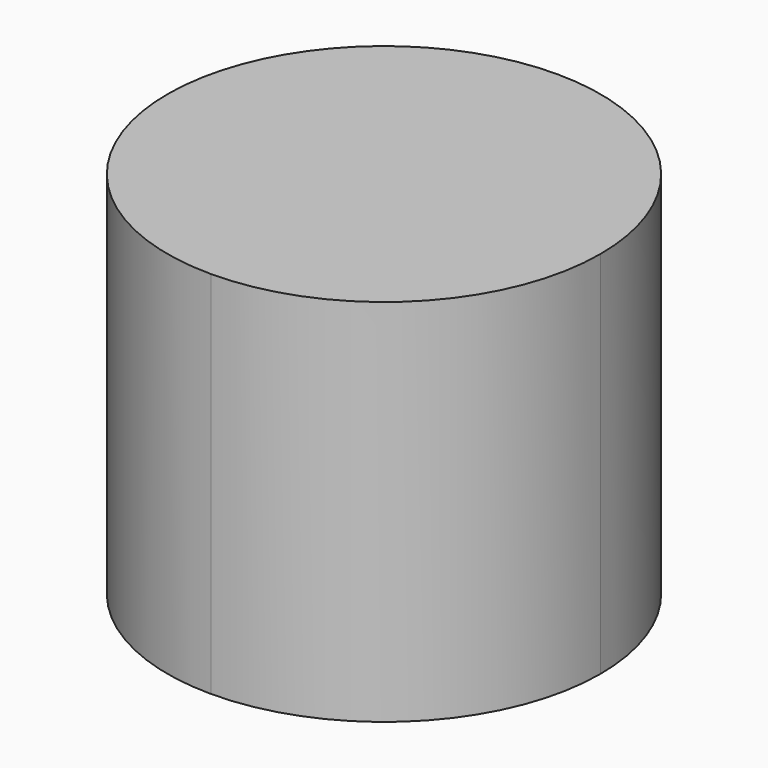
from build123d import *

# Parameters (mm, degrees)
F4_DEPTH = 25.4


# Not quite as in the source:
# - the program builds the solid bodies; features that only make, move or delete a surface that nothing else refers to are left out


with BuildPart() as f4:
    # F2 (on Top) → F4 (new body)
    with BuildSketch(Plane.XY):
        with BuildLine():
            ThreePointArc((0, -14.8716701685), (10.5158588237, -10.5158588237), (14.8716701685, 0))
            ThreePointArc((14.8716701685, 0), (14.0140961938, 4.9771157786), (11.5402781738, 9.3802213871))
            ThreePointArc((11.5402781738, 9.3802213871), (6.390110133, 13.4288147686), (0, 14.8716701685))
            ThreePointArc((0, 14.8716701685), (-6.2616501648, 13.4891923707), (-11.3591281509, 9.598790614))
            ThreePointArc((-11.3591281509, 9.598790614), (-13.9347393829, 5.1951527343), (-14.8705786933, 0.1801747106))
            ThreePointArc((-14.8705786933, 0.1801747106), (-14.0394042685, -4.9052728146), (-11.5226990459, -9.401807289))
            ThreePointArc((-11.5226990459, -9.401807289), (-6.3775385774, -13.4347897377), (0, -14.8716701685))
        make_face()
    extrude(amount=F4_DEPTH)


solid = f4.part
